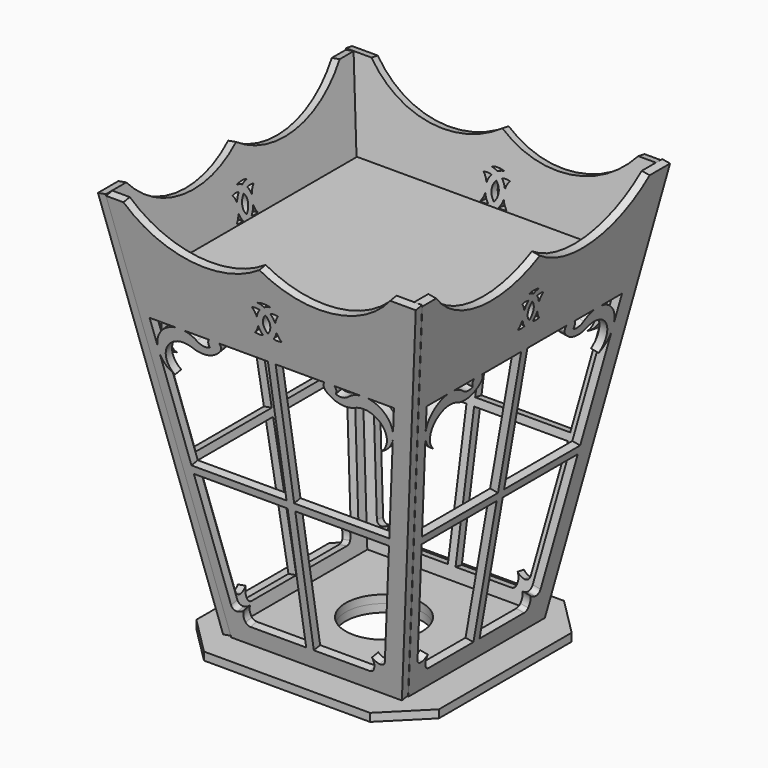
from build123d import *

# Parameters (mm, degrees)
F1_R      = 19.05
F2_DEPTH  = 3.96875
F9_DEPTH  = 3.96875
F11_COUNT = 4
F12_W     = 81.0830884605
F12_H     = 80.8437163355
F12_R     = 19.05
F13_DEPTH = 3.96875
F14_W     = 134.4648289256
F14_H     = 134.4648289256
F15_DEPTH = 3.96875


# Not quite as in the source:
# - a variable given as a bare number and used for a length is read in inches; the dataset says mm whatever the document's units were


with BuildPart() as f2:
    # F1 (on Top) → F2 (new body)
    with BuildSketch(Plane.XY):
        Polygon((60.325, 41.275), (41.275, 60.325), (-41.275, 60.325), (-60.325, 41.275), (-60.325, -41.275), (-41.275, -60.325), (41.275, -60.325), (60.325, -41.275), align=None)
        Circle(F1_R, mode=Mode.SUBTRACT)
    extrude(amount=-F2_DEPTH)


with BuildPart() as f9:
    # F8 (on line) → F9 (new body)
    with BuildSketch(Plane(origin=(0, -43.109668497, -7.6013976854), x_dir=(-1, 0, 0), z_dir=(0, 0.984807753, 0.1736481777))):
        with BuildLine():
            Line((-44.45, 7.7186614973), (40.4218581677, 7.7186614973))
            Line((40.4218581677, 7.7186614973), (75.012751525, 206.9196771487))
            Line((75.012751525, 206.9196771487), (66.3408933573, 206.9196771487))
            ThreePointArc((66.3408933573, 206.9196771487), (34.8985786187, 189.5786347703), (0, 198.0296771487))
            ThreePointArc((0, 198.0296771487), (-34.8985786187, 189.5786347703), (-66.3408933573, 206.9196771487))
            Line((-66.3408933573, 206.9196771487), (-79.0408933573, 206.9196771487))
            Line((-79.0408933573, 206.9196771487), (-44.45, 7.7186614973))
        make_face()
        with BuildLine():
            ThreePointArc((-29.6031839031, 16.6086614973), (-30.9350108228, 16.9858307004), (-31.8713069567, 18.0053252329))
            ThreePointArc((-31.8713069567, 18.0053252329), (-32.5506185367, 20.9332060644), (-31.8073460768, 23.845506948))
            ThreePointArc((-31.8073460768, 23.845506948), (-33.3929100717, 22.6115984826), (-35.2845990495, 21.9348000679))
            ThreePointArc((-35.2845990495, 21.9348000679), (-37.2001021785, 22.345431851), (-38.2536706739, 23.9970262698))
            Line((-38.2536706739, 23.9970262698), (-48.5322784473, 83.189169323))
            Line((-48.5322784473, 83.189169323), (-1.905, 83.189169323))
            Line((-1.905, 83.189169323), (-1.905, 16.6086614973))
            Line((-1.905, 16.6086614973), (-29.6031839031, 16.6086614973))
        make_face(mode=Mode.SUBTRACT)
        with BuildLine():
            ThreePointArc((31.8713069567, 18.0053252329), (30.9350108228, 16.9858307004), (29.6031839031, 16.6086614973))
            Line((29.6031839031, 16.6086614973), (1.905, 16.6086614973))
            Line((1.905, 16.6086614973), (1.905, 83.189169323))
            Line((1.905, 83.189169323), (48.5322784473, 83.189169323))
            Line((48.5322784473, 83.189169323), (38.2536706739, 23.9970262698))
            ThreePointArc((38.2536706739, 23.9970262698), (37.2001021785, 22.345431851), (35.2845990495, 21.9348000679))
            ThreePointArc((35.2845990495, 21.9348000679), (33.3929100717, 22.6115984826), (31.8073460768, 23.845506948))
            ThreePointArc((31.8073460768, 23.845506948), (32.5506185367, 20.9332060644), (31.8713069567, 18.0053252329))
        make_face(mode=Mode.SUBTRACT)
        with BuildLine():
            Line((-58.5279668304, 140.7520445422), (-60.7554618563, 153.5796771487))
            Line((-60.7554618563, 153.5796771487), (-47.7358653811, 153.5796771487))
            ThreePointArc((-47.7358653811, 153.5796771487), (-55.5490123884, 149.1994042977), (-58.5279668304, 140.7520445422))
        make_face(mode=Mode.SUBTRACT)
        with BuildLine():
            Line((-26.1475353943, 153.5796771487), (-1.905, 153.5796771487))
            Line((-1.905, 153.5796771487), (-1.905, 86.999169323))
            Line((-1.905, 86.999169323), (-49.1938780042, 86.999169323))
            Line((-49.1938780042, 86.999169323), (-57.8761220466, 136.9982200421))
            ThreePointArc((-57.8761220466, 136.9982200421), (-55.4084542597, 132.6831137196), (-51.4735058612, 129.6457286631))
            ThreePointArc((-51.4735058612, 129.6457286631), (-53.233586239, 142.8711397112), (-40.3767589249, 146.4364407844))
            ThreePointArc((-40.3767589249, 146.4364407844), (-32.6775135328, 145.6017611026), (-26.1475353943, 149.765227842))
            ThreePointArc((-26.1475353943, 149.765227842), (-25.5108653811, 151.6724524954), (-26.1475353943, 153.5796771487))
        make_face(mode=Mode.SUBTRACT)
        with BuildLine():
            ThreePointArc((-31.2241953678, 153.5796771487), (-31.8608653811, 151.6724524954), (-31.2241953678, 149.765227842))
            ThreePointArc((-31.2241953678, 149.765227842), (-34.5320950878, 149.2973777929), (-37.5758653811, 150.6745294286))
            ThreePointArc((-37.5758653811, 150.6745294286), (-40.5472708831, 152.5721151044), (-43.9258653811, 153.5796771487))
            Line((-43.9258653811, 153.5796771487), (-31.2241953678, 153.5796771487))
        make_face(mode=Mode.SUBTRACT)
        with BuildLine():
            ThreePointArc((-6.5193333333, 165.9506393519), (-5.3192121475, 167.7737343915), (-4.572, 169.8245001974))
            ThreePointArc((-4.572, 169.8245001974), (-3.8247878525, 167.7737343915), (-2.6246666667, 165.9506393519))
            ThreePointArc((-2.6246666667, 165.9506393519), (-4.572, 165.6446771487), (-6.5193333333, 165.9506393519))
        make_face(mode=Mode.SUBTRACT)
        with BuildLine():
            ThreePointArc((-6.5193333333, 178.0387149455), (-4.572, 178.3446771487), (-2.6246666667, 178.0387149455))
            ThreePointArc((-2.6246666667, 178.0387149455), (-3.8247878525, 176.2156199059), (-4.572, 174.1648541))
            ThreePointArc((-4.572, 174.1648541), (-5.3192121475, 176.2156199059), (-6.5193333333, 178.0387149455))
        make_face(mode=Mode.SUBTRACT)
        with BuildLine():
            Line((1.905, 86.999169323), (1.905, 153.5796771487))
            Line((1.905, 153.5796771487), (26.1475353943, 153.5796771487))
            ThreePointArc((26.1475353943, 153.5796771487), (25.5108653811, 151.6724524954), (26.1475353943, 149.765227842))
            ThreePointArc((26.1475353943, 149.765227842), (32.6775135328, 145.6017611026), (40.3767589249, 146.4364407844))
            ThreePointArc((40.3767589249, 146.4364407844), (53.233586239, 142.8711397112), (51.4735058613, 129.6457286631))
            ThreePointArc((51.4735058613, 129.6457286631), (55.4084542597, 132.6831137196), (57.8761220466, 136.9982200421))
            Line((57.8761220466, 136.9982200421), (49.1938780042, 86.999169323))
            Line((49.1938780042, 86.999169323), (1.905, 86.999169323))
        make_face(mode=Mode.SUBTRACT)
        with BuildLine():
            ThreePointArc((43.9258653811, 153.5796771487), (40.5472708831, 152.5721151044), (37.5758653811, 150.6745294286))
            ThreePointArc((37.5758653811, 150.6745294286), (34.5320950878, 149.2973777929), (31.2241953678, 149.7652278421))
            ThreePointArc((31.2241953678, 149.765227842), (31.8608653811, 151.6724524954), (31.2241953678, 153.5796771487))
            Line((31.2241953678, 153.5796771487), (43.9258653811, 153.5796771487))
        make_face(mode=Mode.SUBTRACT)
        with BuildLine():
            Line((47.7358653811, 153.5796771487), (60.7554618563, 153.5796771487))
            Line((60.7554618563, 153.5796771487), (58.5279668304, 140.7520445422))
            ThreePointArc((58.5279668304, 140.7520445422), (55.5490123884, 149.1994042977), (47.7358653811, 153.5796771487))
        make_face(mode=Mode.SUBTRACT)
        with BuildLine():
            ThreePointArc((6.5193333333, 165.9506393519), (4.572, 165.6446771487), (2.6246666667, 165.9506393519))
            ThreePointArc((2.6246666667, 165.9506393519), (3.8247878525, 167.7737343915), (4.572, 169.8245001974))
            ThreePointArc((4.572, 169.8245001974), (5.3192121475, 167.7737343915), (6.5193333333, 165.9506393519))
        make_face(mode=Mode.SUBTRACT)
        with BuildLine():
            ThreePointArc((0, 167.5879418492), (-1.778, 171.9946771487), (0, 176.4014124482))
            ThreePointArc((0, 176.4014124482), (1.778, 171.9946771487), (0, 167.5879418492))
        make_face(mode=Mode.SUBTRACT)
        with BuildLine():
            ThreePointArc((3.175, 181.2882660679), (1.5388032001, 180.8897387659), (0, 180.2055979253))
            ThreePointArc((0, 180.2055979253), (-1.5388032001, 180.8897387659), (-3.175, 181.2882660679))
            ThreePointArc((-3.175, 181.2882660679), (0, 181.8156455327), (3.175, 181.2882660679))
        make_face(mode=Mode.SUBTRACT)
        with BuildLine():
            ThreePointArc((2.6246666667, 178.0387149455), (4.572, 178.3446771487), (6.5193333333, 178.0387149455))
            ThreePointArc((6.5193333333, 178.0387149455), (5.3192121475, 176.2156199059), (4.572, 174.1648541))
            ThreePointArc((4.572, 174.1648541), (3.8247878525, 176.2156199059), (2.6246666667, 178.0387149455))
        make_face(mode=Mode.SUBTRACT)
    extrude(amount=F9_DEPTH)


with BuildPart() as f11_1:
    # F11: instance of F9
    add(f9.part.rotate(Axis((0, 0, 65.0201365352), (0, 0, 1)), 1 * 360 / F11_COUNT))


with BuildPart() as f11_2:
    # F11: instance of F9
    add(f9.part.rotate(Axis((0, 0, 65.0201365352), (0, 0, 1)), 2 * 360 / F11_COUNT))


with BuildPart() as f11_3:
    # F11: instance of F9
    add(f9.part.rotate(Axis((0, 0, 65.0201365352), (0, 0, 1)), 3 * 360 / F11_COUNT))


with BuildPart() as f13:
    # F12 (on Top) → F13 (new body)
    with BuildSketch(Plane.XY):
        Rectangle(F12_W, F12_H)
        Circle(F12_R, mode=Mode.SUBTRACT)
    extrude(amount=F13_DEPTH)


with BuildPart() as f15:
    # F14 (on offset) → F15 (new body)
    with BuildSketch(Plane.XY.offset(152.4)):
        with Locations((0.0598430312, -0.0598430312)):
            Rectangle(F14_W, F14_H)
    extrude(amount=F15_DEPTH)


solid = Compound([f2.part, f9.part, f11_1.part, f11_2.part, f11_3.part, f13.part, f15.part])
